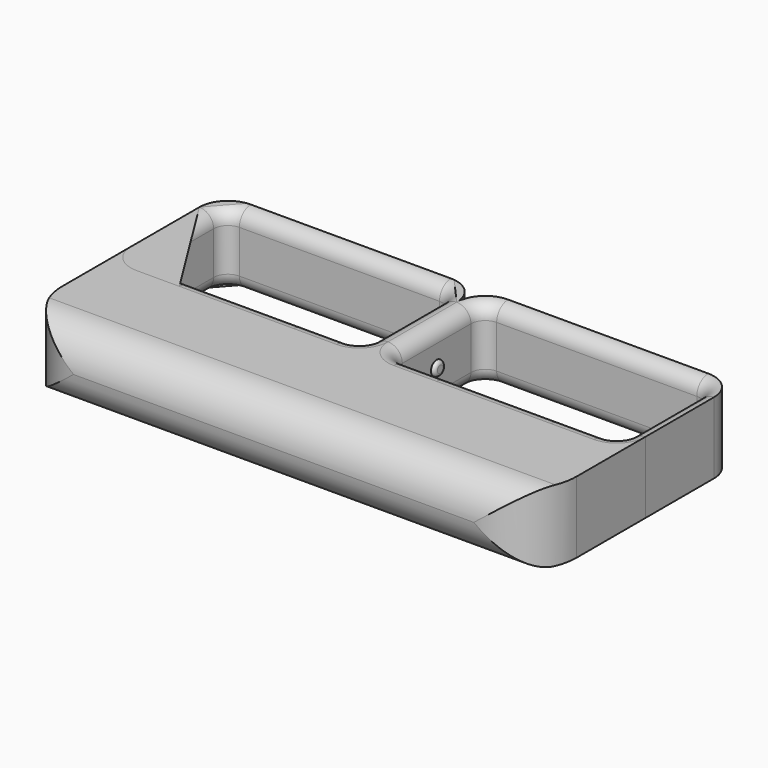
from build123d import *

# Parameters (mm, degrees)
F1_DEPTH      = 15.875
F3_DEPTH      = 15.875
F4_R          = 1.5875
F5_DEPTH      = 3.96875
F5_DEPTH_BACK = 3.96875
F6_R          = 0.79374
F7_R          = 1.5875
F8_DEPTH      = 22.225
F8_DEPTH_BACK = 4.7625
F9_R          = 1.58749
F10_T1_DEPTH  = 128.5875
F11_R         = 3.17499
F11_2_R       = 3.17499


# Not quite as in the source:
# - a fillet or chamfer that OpenCascade refuses, or shapes differently, is made with other operations: its cross-section is extruded or revolved along the edge and cut away or added
# - a fillet or chamfer is up to 0.001 mm smaller than in the source, because OpenCascade refuses the exact size


with BuildPart() as f1:
    # F0 (on Top) → F1 (new body)
    with BuildSketch(Plane.XY):
        with BuildLine():
            Line((-15.875, 0), (-6.35, 0))
            ThreePointArc((-6.35, 0), (-1.8598719395, 1.8598719395), (0, 6.35))
            Line((0, 6.35), (0, 25.4))
            ThreePointArc((0, 25.4), (-1.8598719395, 29.8901280605), (-6.35, 31.75))
            Line((-6.35, 31.75), (-50.8, 31.75))
            ThreePointArc((-50.8, 31.75), (-55.2901280605, 29.8901280605), (-57.15, 25.4))
            Line((-57.15, 25.4), (-57.15, 6.35))
            ThreePointArc((-57.15, 6.35), (-55.2901280605, 1.8598719395), (-50.8, 0))
            Line((-50.8, 0), (-41.275, 0))
            Line((-41.275, 0), (-41.275, 3.175))
            Line((-41.275, 3.175), (-50.8, 3.175))
            ThreePointArc((-50.8, 3.175), (-53.0450640303, 4.1049359697), (-53.975, 6.35))
            Line((-53.975, 6.35), (-53.975, 25.4))
            ThreePointArc((-53.975, 25.4), (-53.0450640303, 27.6450640303), (-50.8, 28.575))
            Line((-50.8, 28.575), (-6.35, 28.575))
            ThreePointArc((-6.35, 28.575), (-4.1049359697, 27.6450640303), (-3.175, 25.4))
            Line((-3.175, 25.4), (-3.175, 6.35))
            ThreePointArc((-3.175, 6.35), (-4.1049359697, 4.1049359697), (-6.35, 3.175))
            Line((-6.35, 3.175), (-15.875, 3.175))
            Line((-15.875, 3.175), (-15.875, 0))
        make_face()
        with BuildLine():
            Line((0, 25.4), (0, 6.35))
            ThreePointArc((0, 6.35), (1.8598719395, 1.8598719395), (6.35, 0))
            Line((6.35, 0), (15.875, 0))
            Line((15.875, 0), (15.875, 3.175))
            Line((15.875, 3.175), (6.35, 3.175))
            ThreePointArc((6.35, 3.175), (4.1049359697, 4.1049359697), (3.175, 6.35))
            Line((3.175, 6.35), (3.175, 25.4))
            ThreePointArc((3.175, 25.4), (4.1049359697, 27.6450640303), (6.35, 28.575))
            Line((6.35, 28.575), (50.8, 28.575))
            ThreePointArc((50.8, 28.575), (53.0450640303, 27.6450640303), (53.975, 25.4))
            Line((53.975, 25.4), (53.975, 6.35))
            ThreePointArc((53.975, 6.35), (53.0450640303, 4.1049359697), (50.8, 3.175))
            Line((50.8, 3.175), (41.275, 3.175))
            Line((41.275, 3.175), (41.275, 0))
            Line((41.275, 0), (50.8, 0))
            ThreePointArc((50.8, 0), (55.2901280605, 1.8598719395), (57.15, 6.35))
            Line((57.15, 6.35), (57.15, 25.4))
            ThreePointArc((57.15, 25.4), (55.2901280605, 29.8901280605), (50.8, 31.75))
            Line((50.8, 31.75), (6.35, 31.75))
            ThreePointArc((6.35, 31.75), (1.8598719395, 29.8901280605), (0, 25.4))
        make_face()
    extrude(amount=F1_DEPTH)

    # F4 (on Right) → F5 (join, two sides)
    with BuildSketch(Plane.YZ) as f5_sk:
        with Locations((15.875, 7.9375)):
            Circle(F4_R)
    extrude(amount=F5_DEPTH)
    extrude(f5_sk.sketch, amount=-F5_DEPTH_BACK)

    # F6 (radius 0.79375 in the source; OpenCascade refuses exactly that, so slightly less here)
    f6_edges = [f1.edges().sort_by_distance(p)[0] for p in [
        (-3.96875, 14.2875, 7.9375),
        (3.96875, 14.2875, 7.9375),
    ]]
    fillet(f6_edges, radius=F6_R)

    # F7 (on Front) → F8 (join, two sides)
    with BuildSketch(Plane.XZ) as f8_sk:
        with Locations((-9.525, 7.9375)):
            Circle(F7_R)
        with Locations((9.525, 7.9375)):
            Circle(F7_R)
        with Locations((-47.625, 7.9375)):
            Circle(F7_R)
        with Locations((47.625, 7.9375)):
            Circle(F7_R)
    extrude(amount=F8_DEPTH)
    extrude(f8_sk.sketch, amount=-F8_DEPTH_BACK)

    # F9 (radius 1.5875 in the source; OpenCascade refuses exactly that, so slightly less here)
    f9_edges = [f1.edges().sort_by_distance(p)[0] for p in [
        (46.0375, 4.7625, 7.9375),
        (7.9375, 4.7625, 7.9375),
        (-11.1125, 4.7625, 7.9375),
        (-49.2125, 4.7625, 7.9375),
    ]]
    fillet(f9_edges, radius=F9_R)

    # F11 (radius 3.175 in the source; OpenCascade refuses exactly that, so slightly less here)
    f11_edges = [f1.edges().sort_by_distance(p)[0] for p in [
        (11.1125, 3.175, 15.875),
        (11.1125, 3.175, 0),
        (46.0375, 3.175, 0),
        (46.0375, 3.175, 15.875),
        (-11.1125, 3.175, 0),
        (-11.1125, 3.175, 15.875),
        (-46.0375, 3.175, 15.875),
        (-46.0375, 3.175, 0),
        (-4.104936, 4.104936, 0),
        (-3.175, 15.875, 0),
        (-3.175, 15.875, 15.875),
        (-4.104936, 4.104936, 15.875),
        (3.175, 15.875, 0),
        (3.175, 15.875, 15.875),
        (4.104936, 4.104936, 0),
        (4.104936, 4.104936, 15.875),
        (4.104936, 27.645064, 0),
        (28.575, 28.575, 0),
        (53.045064, 27.645064, 0),
        (53.975, 15.875, 0),
        (53.045064, 4.104936, 0),
        (-53.045064, 4.104936, 0),
        (-53.975, 15.875, 0),
        (-53.045064, 27.645064, 0),
        (-28.575, 28.575, 0),
        (-4.104936, 27.645064, 0),
        (4.104936, 27.645064, 15.875),
        (28.575, 28.575, 15.875),
        (53.045064, 27.645064, 15.875),
        (53.975, 15.875, 15.875),
        (53.045064, 4.104936, 15.875),
        (-53.045064, 4.104936, 15.875),
        (-53.975, 15.875, 15.875),
        (-53.045064, 27.645064, 15.875),
        (-28.575, 28.575, 15.875),
        (-4.104936, 27.645064, 15.875),
    ]]
    fillet(f11_edges, radius=F11_R)


with BuildPart() as f3:
    # F2 (on Top) → F3 (new body)
    with BuildSketch(Plane.XY):
        with BuildLine():
            ThreePointArc((57.15, 6.35), (55.2901280605, 1.8598719395), (50.8, 0))
            Line((50.8, 0), (41.275, 0))
            Line((41.275, 0), (41.275, 3.175))
            Line((41.275, 3.175), (15.875, 3.175))
            Line((15.875, 3.175), (15.875, 0))
            Line((15.875, 0), (6.35, 0))
            ThreePointArc((6.35, 0), (1.8598719395, 1.8598719395), (0, 6.35))
            ThreePointArc((0, 6.35), (-1.8598719395, 1.8598719395), (-6.35, 0))
            Line((-6.35, 0), (-15.875, 0))
            Line((-15.875, 0), (-15.875, 3.175))
            Line((-15.875, 3.175), (-41.275, 3.175))
            Line((-41.275, 3.175), (-41.275, 0))
            Line((-41.275, 0), (-50.8, 0))
            ThreePointArc((-50.8, 0), (-55.2901280605, 1.8598719395), (-57.15, 6.35))
            Line((-57.15, 6.35), (-57.15, 0))
            Line((-57.15, 0), (-57.15, -12.7))
            ThreePointArc((-57.15, -12.7), (-53.4302561211, -21.6802561211), (-44.45, -25.4))
            Line((-44.45, -25.4), (44.45, -25.4))
            ThreePointArc((44.45, -25.4), (53.4302561211, -21.6802561211), (57.15, -12.7))
            Line((57.15, -12.7), (57.15, 0))
            Line((57.15, 0), (57.15, 6.35))
        make_face()
    extrude(amount=F3_DEPTH)

    # F10: fillet of radius 7.9375 on 2 edges, made by hand

    # F10_s2 → F10_t1 (cut)
    with BuildSketch(Plane.YZ.offset(-64.29375)):
        with BuildLine():
            ThreePointArc((-17.4625, 15.875), (-23.0751600757, 13.5501600757), (-25.4, 7.9375))
            Line((-25.4, 7.9375), (-25.4, 15.875))
            Line((-25.4, 15.875), (-17.4625, 15.875))
        make_face()
        with BuildLine():
            ThreePointArc((-25.4, 7.9375), (-23.0751600757, 2.3248399243), (-17.4625, 0))
            Line((-17.4625, 0), (-25.4, 0))
            Line((-25.4, 0), (-25.4, 7.9375))
        make_face()
    extrude(amount=F10_T1_DEPTH, mode=Mode.SUBTRACT)

    # F11#2 (radius 3.175 in the source; OpenCascade refuses exactly that, so slightly less here)
    f11_2_edges = [f3.edges().sort_by_distance(p)[0] for p in [
        (-28.575, 3.175, 0),
        (-28.575, 3.175, 15.875),
        (28.575, 3.175, 0),
        (28.575, 3.175, 15.875),
    ]]
    fillet(f11_2_edges, radius=F11_2_R)


solid = Compound([f1.part, f3.part])
